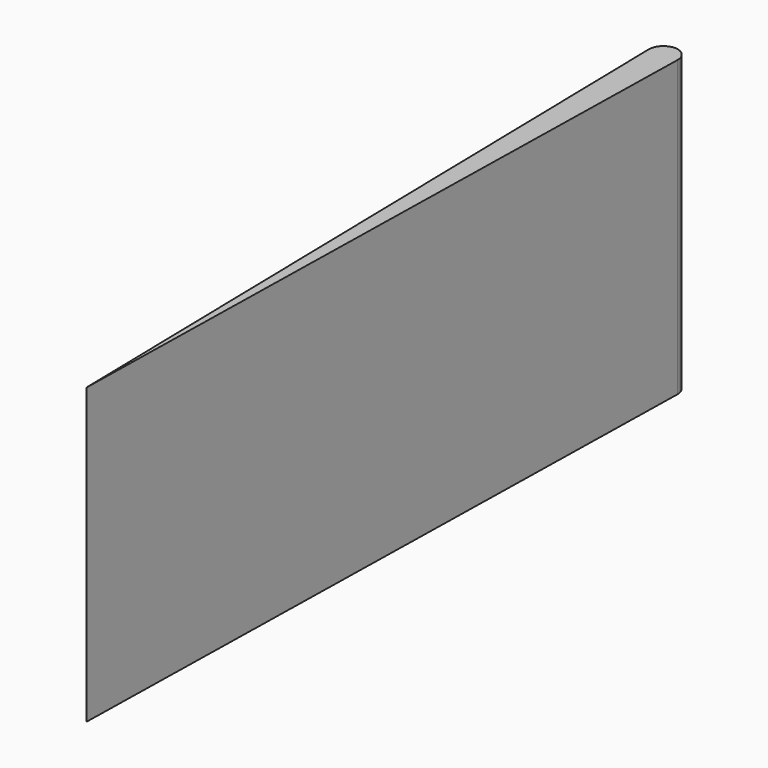
from build123d import *

# Parameters (mm, degrees)
F1_DEPTH    = 40
F2_T1_DEPTH = 50.2019998


# Not quite as in the source:
# - a fillet or chamfer that OpenCascade refuses, or shapes differently, is made with other operations: its cross-section is extruded or revolved along the edge and cut away or added


with BuildPart() as f1:
    # F0 (on Top) → F1 (new body)
    with BuildSketch(Plane.XY):
        Polygon((2, 0), (0, 0), (-2, 0), (0, -100), align=None)
    extrude(amount=F1_DEPTH)

    # F2: fillet of radius 2 on 2 edges, made by hand

    # F2_s2 → F2_t1 (cut)
    with BuildSketch(Plane.XY.offset(-5.1009999)):
        with BuildLine():
            ThreePointArc((0.04039996, 0), (-1.387882926, -0.5999971437), (-1.95920016, -2.0399920024))
            Line((-1.95920016, -2.0399920024), (-2, 0))
            Line((-2, 0), (0.04039996, 0))
        make_face()
        with BuildLine():
            ThreePointArc((-0.04039996, 0), (1.387882926, -0.5999971437), (1.95920016, -2.0399920024))
            Line((1.95920016, -2.0399920024), (2, 0))
            Line((2, 0), (-0.04039996, 0))
        make_face()
    extrude(amount=F2_T1_DEPTH, mode=Mode.SUBTRACT)


solid = f1.part
